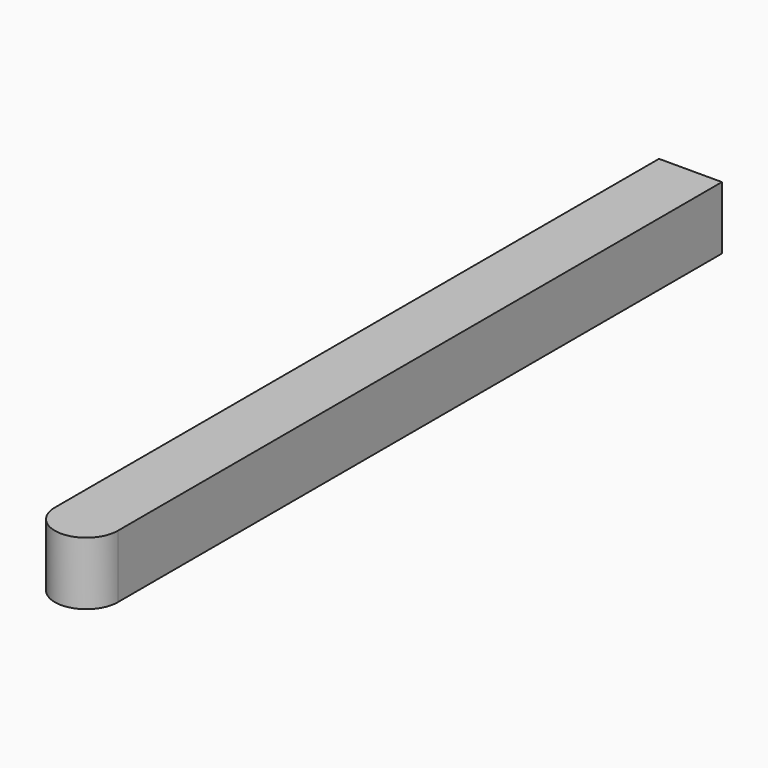
from build123d import *

# Parameters (mm, degrees)
F1_DEPTH = 1.5875


with BuildPart() as f1:
    # F0 (on Top) → F1 (new body)
    with BuildSketch(Plane.XY):
        with BuildLine():
            Line((-63.5, 31.75), (-64.29375, 31.75))
            Line((-64.29375, 31.75), (-64.29375, 12.7))
            ThreePointArc((-64.29375, 12.7), (-63.5, 11.90625), (-62.70625, 12.7))
            Line((-62.70625, 12.7), (-62.70625, 31.75))
            Line((-62.70625, 31.75), (-63.5, 31.75))
        make_face()
    extrude(amount=F1_DEPTH)


solid = f1.part
